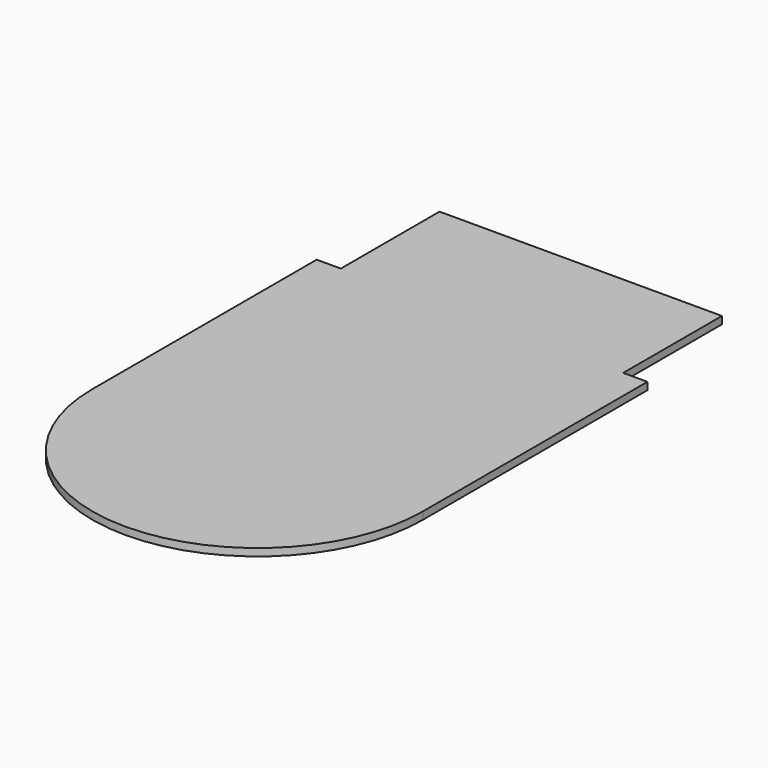
from build123d import *

# Parameters (mm, degrees)
F1_DEPTH = 1


# Not quite as in the source:
# - a feature names something its author has since deleted; it is built from what else it names


with BuildPart() as f1:
    # F0 (on Top) → F1 (new body)
    with BuildSketch(Plane.XY):
        with BuildLine():
            Line((-19, 37.75), (-22.25, 37.75))
            Line((-22.25, 37.75), (-22.25, 0))
            ThreePointArc((-22.25, 0), (0, -22.25), (22.25, 0))
            Line((22.25, 0), (22.25, 37.75))
            Line((22.25, 37.75), (19, 37.75))
            Line((19, 37.75), (19, 54.3464050591))
            Line((19, 54.3464050591), (-19, 54.3464050591))
            Line((-19, 54.3464050591), (-19, 42.75))
            Line((-19, 42.75), (-19, 37.75))
        make_face()
    extrude(amount=F1_DEPTH)


solid = f1.part
